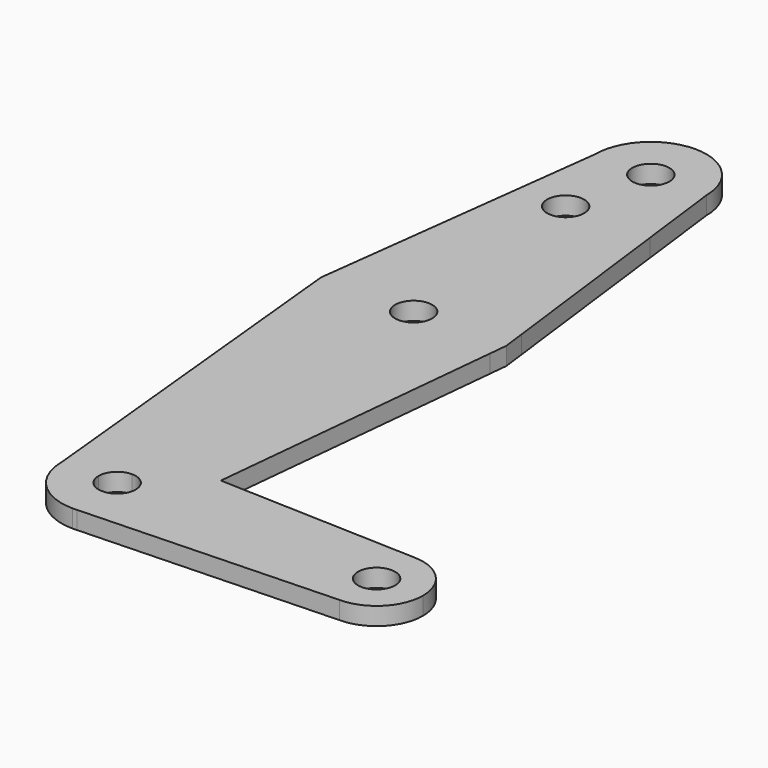
from build123d import *

# Parameters (mm, degrees)
F0_R     = 3.175
F1_DEPTH = 3.048


with BuildPart() as f1:
    # F0 (on Top) → F1 (new body)
    with BuildSketch(Plane.XY):
        with BuildLine():
            ThreePointArc((-36.1690279353, 68.7742138668), (-26.6440279353, 59.2492138668), (-17.1190279353, 68.7742138668))
            ThreePointArc((-17.1190279353, 68.7742138668), (-26.6440279353, 78.2992138668), (-36.1690279353, 68.7742138668))
        make_face()
        with Locations((-26.6440279353, 68.7742138668)):
            Circle(F0_R, mode=Mode.SUBTRACT)
        with BuildLine():
            Line((-15.3346779353, 54.4994138668), (-17.1190279353, 68.7742138668))
            ThreePointArc((-17.1190279353, 68.7742138668), (-26.6440279353, 59.2492138668), (-36.1690279353, 68.7742138668))
            Line((-36.1690279353, 68.7742138668), (-42.0305663969, 21.8819061745))
            ThreePointArc((-42.0305663969, 21.8819061745), (-26.6440279353, 33.8492138668), (-11.2574894738, 21.8819061745))
            Line((-11.2574894738, 21.8819061745), (-15.3346779353, 54.4994138668))
        make_face()
        with Locations((-29.8190279353, 54.4994138668)):
            Circle(F0_R, mode=Mode.SUBTRACT)
        with BuildLine():
            ThreePointArc((-11.2574894738, 21.8819061745), (-26.6440279353, 33.8492138668), (-42.0305663969, 21.8819061745))
            Line((-42.0305663969, 21.8819061745), (-42.5190279353, 17.9742138668))
            Line((-42.5190279353, 17.9742138668), (-42.2046714997, 14.8306495103))
            ThreePointArc((-42.2046714997, 14.8306495103), (-26.6440279353, 2.0992138668), (-11.083384371, 14.8306495103))
            Line((-11.083384371, 14.8306495103), (-10.7690279353, 17.9742138668))
            Line((-10.7690279353, 17.9742138668), (-11.2574894738, 21.8819061745))
        make_face()
        with Locations((-26.6440279353, 17.9742138668)):
            Circle(F0_R, mode=Mode.SUBTRACT)
        with BuildLine():
            ThreePointArc((-11.083384371, 14.8306495103), (-26.6440279353, 2.0992138668), (-42.2046714997, 14.8306495103))
            Line((-42.2046714997, 14.8306495103), (-36.1690279353, -45.5257861332))
            ThreePointArc((-36.1690279353, -45.5257861332), (-33.3792200261, -38.7905940424), (-26.6440279353, -36.0007861332))
            ThreePointArc((-26.6440279353, -36.0007861332), (-26.3040661072, -36.0068549456), (-25.9645374895, -36.0250536492))
            Line((-25.9645374895, -36.0250536492), (-16.2038144122, -36.3736509019))
            Line((-16.2038144122, -36.3736509019), (-11.083384371, 14.8306495103))
        make_face()
        with BuildLine():
            Line((-29.8190279353, -45.5257861332), (-36.1690279353, -45.5257861332))
            ThreePointArc((-36.1690279353, -45.5257861332), (-33.3792200261, -52.260978224), (-26.6440279353, -55.0507861332))
            Line((-26.6440279353, -55.0507861332), (-25.9645374895, -55.0265186173))
            ThreePointArc((-25.9645374895, -55.0265186173), (-19.6727378289, -52.0162976117), (-17.1190279353, -45.5257861332))
            Line((-17.1190279353, -45.5257861332), (-23.4690279353, -45.5257861332))
            ThreePointArc((-23.4690279353, -45.5257861332), (-26.6440279353, -48.7007861332), (-29.8190279353, -45.5257861332))
        make_face()
        with BuildLine():
            ThreePointArc((-26.6440279353, -36.0007861332), (-33.3792200261, -38.7905940424), (-36.1690279353, -45.5257861332))
            Line((-36.1690279353, -45.5257861332), (-29.8190279353, -45.5257861332))
            ThreePointArc((-29.8190279353, -45.5257861332), (-28.8890919656, -43.280722103), (-26.6440279353, -42.3507861332))
            Line((-26.6440279353, -42.3507861332), (-26.6440279353, -36.0007861332))
        make_face()
        with BuildLine():
            Line((17.8059720647, -37.5882861332), (-16.2038144122, -36.3736509019))
            Line((-16.2038144122, -36.3736509019), (-17.1190279353, -45.5257861332))
            ThreePointArc((-17.1190279353, -45.5257861332), (-19.6727378289, -52.0162976117), (-25.9645374895, -55.0265186173))
            Line((-25.9645374895, -55.0265186173), (17.8059720647, -53.4632861332))
            ThreePointArc((17.8059720647, -53.4632861332), (12.193311989, -51.1384462089), (9.8684720647, -45.5257861332))
            ThreePointArc((9.8684720647, -45.5257861332), (12.193311989, -39.9131260576), (17.8059720647, -37.5882861332))
        make_face()
        with BuildLine():
            Line((-17.1190279353, -45.5257861332), (-16.2038144122, -36.3736509019))
            Line((-16.2038144122, -36.3736509019), (-25.9645374895, -36.0250536492))
            ThreePointArc((-25.9645374895, -36.0250536492), (-19.6727378289, -39.0352746548), (-17.1190279353, -45.5257861332))
        make_face()
        with BuildLine():
            Line((-25.9645374895, -36.0250536492), (-26.6440279353, -36.0007861332))
            Line((-26.6440279353, -36.0007861332), (-26.6440279353, -42.3507861332))
            ThreePointArc((-26.6440279353, -42.3507861332), (-24.3989639051, -43.280722103), (-23.4690279353, -45.5257861332))
            Line((-23.4690279353, -45.5257861332), (-17.1190279353, -45.5257861332))
            ThreePointArc((-17.1190279353, -45.5257861332), (-19.6727378289, -39.0352746548), (-25.9645374895, -36.0250536492))
        make_face()
        with BuildLine():
            ThreePointArc((25.7434720647, -45.5257861332), (23.4186321403, -39.9131260576), (17.8059720647, -37.5882861332))
            ThreePointArc((17.8059720647, -37.5882861332), (12.193311989, -39.9131260576), (9.8684720647, -45.5257861332))
            Line((9.8684720647, -45.5257861332), (14.6309720647, -45.5257861332))
            ThreePointArc((14.6309720647, -45.5257861332), (17.8059720647, -42.3507861332), (20.9809720647, -45.5257861332))
            Line((20.9809720647, -45.5257861332), (25.7434720647, -45.5257861332))
        make_face()
        with BuildLine():
            ThreePointArc((17.8059720647, -53.4632861332), (23.4186321403, -51.1384462089), (25.7434720647, -45.5257861332))
            Line((25.7434720647, -45.5257861332), (20.9809720647, -45.5257861332))
            ThreePointArc((20.9809720647, -45.5257861332), (17.8059720647, -48.7007861332), (14.6309720647, -45.5257861332))
            Line((14.6309720647, -45.5257861332), (9.8684720647, -45.5257861332))
            ThreePointArc((9.8684720647, -45.5257861332), (12.193311989, -51.1384462089), (17.8059720647, -53.4632861332))
        make_face()
    extrude(amount=F1_DEPTH)


solid = f1.part
